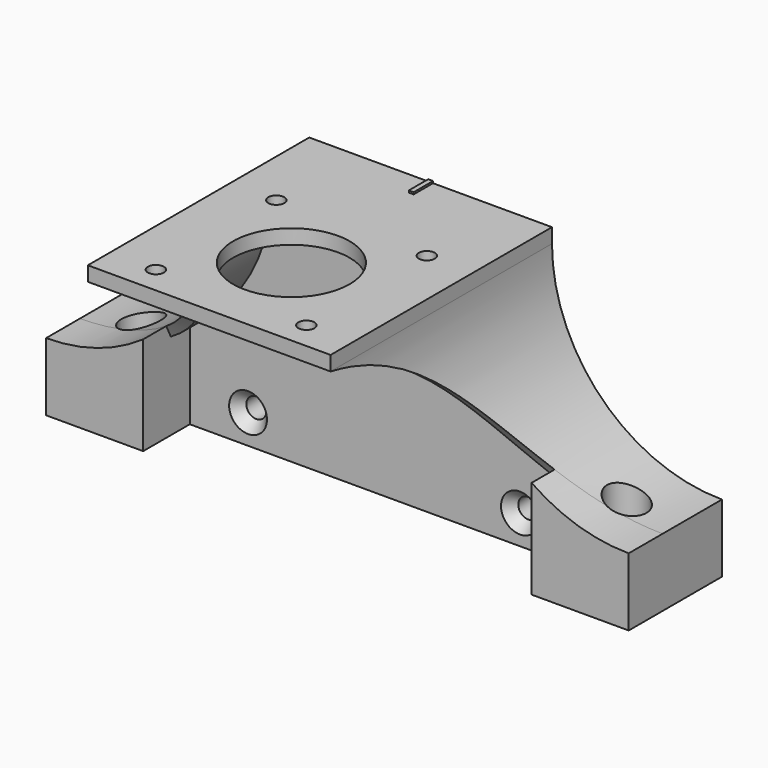
from build123d import *

# Parameters (mm, degrees)
F0_W           = 50
F0_H           = 3
F1_DEPTH       = 12
F3_DEPTH       = 45
F5_DEPTH       = 120.001
F6_R           = 12
F6_R_2         = 1.65
F7_DEPTH       = 25
F9_D           = 4.1000000042
F9_CSINK_D     = 7.7978
F9_CSINK_ANGLE = 82
F10_W          = 1
F10_H          = 5
F11_DEPTH      = 0.4
F13_END_RADIUS = 35
F13_REACH      = 75.7248075794
F14_END_RADIUS = 35
F14_REACH      = 75.7248075794
F15_DEPTH      = 25


with BuildPart() as f1:
    # F0 (on Front) → F1 (new body)
    with BuildSketch(Plane.XZ):
        with BuildLine():
            Line((22.8227958083, 19.723181963), (-27.1772041917, 19.723181963))
            ThreePointArc((-27.1772041917, 19.723181963), (-37.4284668502, -5.0255553786), (-62.1772041917, -15.276818037))
            Line((-62.1772041917, -15.276818037), (-62.1772041917, -29.276818037))
            Line((-62.1772041917, -29.276818037), (57.8227958083, -29.276818037))
            Line((57.8227958083, -29.276818037), (57.8227958083, -15.276818037))
            ThreePointArc((57.8227958083, -15.276818037), (33.0740584668, -5.0255553786), (22.8227958083, 19.723181963))
        make_face()
        with Locations((-2.1772041917, 21.223181963)):
            Rectangle(F0_W, F0_H)
    extrude(amount=F1_DEPTH)

    # F2 (on face) → F3 (join)
    with BuildSketch(Plane.XZ.offset(12)):
        with BuildLine():
            Line((-25.1772041917, 19.723181963), (-27.1772041917, 19.723181963))
            ThreePointArc((-27.1772041917, 19.723181963), (-37.4284668502, -5.0255553786), (-62.1772041917, -15.276818037))
            Line((-62.1772041917, -15.276818037), (-62.1772041917, -29.276818037))
            Line((-62.1772041917, -29.276818037), (-60.1772041917, -29.276818037))
            Line((-60.1772041917, -29.276818037), (-60.1772041917, -17.2227244409))
            ThreePointArc((-60.1772041917, -17.2227244409), (-35.3164521546, -5.722839337), (-25.1772041917, 19.723181963))
        make_face()
        Polygon((-27.1772041917, 22.723181963), (-27.1772041917, 19.723181963), (-25.1772041917, 19.723181963), (20.8227958083, 19.723181963), (22.8227958083, 19.723181963), (22.8227958083, 22.723181963), align=None)
        with BuildLine():
            Line((22.8227958083, 19.723181963), (20.8227958083, 19.723181963))
            ThreePointArc((20.8227958083, 19.723181963), (30.9620437712, -5.722839337), (55.8227958083, -17.2227244409))
            Line((55.8227958083, -17.2227244409), (55.8227958083, -29.276818037))
            Line((55.8227958083, -29.276818037), (57.8227958083, -29.276818037))
            Line((57.8227958083, -29.276818037), (57.8227958083, -15.276818037))
            ThreePointArc((57.8227958083, -15.276818037), (33.0740584668, -5.0255553786), (22.8227958083, 19.723181963))
        make_face()
    extrude(amount=F3_DEPTH)

    # F4 (on face) → F5 (cut, through all)
    with BuildSketch(Plane(origin=(-62.1772041917, 0, 0), x_dir=(0, -1, 0), z_dir=(-1, 0, 0))):
        with BuildLine():
            Line((57, -15.276818037), (57, 19.723181963))
            ThreePointArc((57, 19.723181963), (26.3280584166, 2.7280262742), (12, -29.276818037))
            Line((12, -29.276818037), (57, -29.276818037))
            Line((57, -29.276818037), (57, -15.276818037))
        make_face()
    extrude(amount=-F5_DEPTH, mode=Mode.SUBTRACT)

    # F6 (on face) → F7 (cut)
    with BuildSketch(Plane.XY.offset(22.723181963)):
        with Locations((-2.1772041917, -35.85)):
            Circle(F6_R)
        with Locations((-17.6772041917, -51.35)):
            Circle(F6_R_2)
        with Locations((-17.6772041917, -20.35)):
            Circle(F6_R_2)
        with Locations((13.3227958083, -51.35)):
            Circle(F6_R_2)
        with Locations((13.3227958083, -20.35)):
            Circle(F6_R_2)
    extrude(amount=-F7_DEPTH, mode=Mode.SUBTRACT)

    # F9 (through all)
    with Locations(Plane.XZ.offset(12)):
        with Locations((-30.1772041917, -23.2497712389), (25.8227958083, -23.2497712389)):
            CounterSinkHole(F9_D / 2, F9_CSINK_D / 2, counter_sink_angle=F9_CSINK_ANGLE)

    # F10 (on face) → F11 (join)
    with BuildSketch(Plane.XY.offset(22.723181963)):
        with Locations((-2.1772041917, -2.5)):
            Rectangle(F10_W, F10_H)
    extrude(amount=F11_DEPTH)

    f13_end = (Plane(origin=(-62.1772041917, -28.5, 19.723181963), x_dir=(0, 0, 1), z_dir=(0, 1, 0)) * Cylinder(F13_END_RADIUS, 437.0700631752, mode=Mode.PRIVATE)).faces().sort_by_distance((-37.4284668502, -0.7549172174, -5.0255553786))[0]
    # F12 (on face) → F13 (join, up to the whole of a round face its end follows)
    with BuildSketch(Plane(origin=(0, 0, -29.276818037), x_dir=(1, 0, 0), z_dir=(0, 0, -1))):
        with BuildLine():
            Line((-62.1772041917, 24), (-62.1772041917, 12))
            Line((-62.1772041917, 12), (-60.1772041917, 12))
            Line((-60.1772041917, 12), (-56.2272041917, 12))
            ThreePointArc((-56.2272041917, 12), (-52.1772041917, 16.05), (-48.1272041917, 12))
            Line((-48.1272041917, 12), (-42.1772041917, 12))
            Line((-42.1772041917, 12), (-42.1772041917, 24))
            Line((-42.1772041917, 24), (-62.1772041917, 24))
        make_face()
        with BuildLine():
            Line((-56.2272041917, 12), (-48.1272041917, 12))
            ThreePointArc((-48.1272041917, 12), (-52.1772041917, 16.05), (-56.2272041917, 12))
        make_face()
    f13_long = extrude(amount=-F13_REACH, mode=Mode.PRIVATE)
    add(split(f13_long, bisect_by=f13_end, keep=Keep.TOP, mode=Mode.PRIVATE))

    f14_end = (Plane(origin=(57.8227958083, -28.5, 19.723181963), x_dir=(0, 0, 1), z_dir=(0, 1, 0)) * Cylinder(F14_END_RADIUS, 437.0700631752, mode=Mode.PRIVATE)).faces().sort_by_distance((33.0740584668, -0.7549172174, -5.0255553786))[0]
    # F12 (on face) → F14 (join, up to the whole of a round face its end follows)
    with BuildSketch(Plane(origin=(0, 0, -29.276818037), x_dir=(1, 0, 0), z_dir=(0, 0, -1))):
        with BuildLine():
            Line((37.8227958083, 24), (37.8227958083, 12))
            Line((37.8227958083, 12), (43.7727958083, 12))
            ThreePointArc((43.7727958083, 12), (47.8227958083, 16.05), (51.8727958083, 12))
            Line((51.8727958083, 12), (55.8227958083, 12))
            Line((55.8227958083, 12), (57.8227958083, 12))
            Line((57.8227958083, 12), (57.8227958083, 24))
            Line((57.8227958083, 24), (37.8227958083, 24))
        make_face()
        with BuildLine():
            Line((51.8727958083, 12), (43.7727958083, 12))
            ThreePointArc((43.7727958083, 12), (47.8227958083, 7.95), (51.8727958083, 12))
        make_face()
    f14_long = extrude(amount=-F14_REACH, mode=Mode.PRIVATE)
    add(split(f14_long, bisect_by=f14_end, keep=Keep.TOP, mode=Mode.PRIVATE))

    # F12 (on face) → F15 (cut)
    with BuildSketch(Plane(origin=(0, 0, -29.276818037), x_dir=(1, 0, 0), z_dir=(0, 0, -1))):
        with BuildLine():
            Line((-56.2272041917, 12), (-48.1272041917, 12))
            ThreePointArc((-48.1272041917, 12), (-52.1772041917, 16.05), (-56.2272041917, 12))
        make_face()
        with BuildLine():
            ThreePointArc((-56.2272041917, 12), (-52.1772041917, 7.95), (-48.1272041917, 12))
            Line((-48.1272041917, 12), (-56.2272041917, 12))
        make_face()
        with BuildLine():
            Line((51.8727958083, 12), (43.7727958083, 12))
            ThreePointArc((43.7727958083, 12), (47.8227958083, 7.95), (51.8727958083, 12))
        make_face()
        with BuildLine():
            ThreePointArc((51.8727958083, 12), (47.8227958083, 16.05), (43.7727958083, 12))
            Line((43.7727958083, 12), (51.8727958083, 12))
        make_face()
    extrude(amount=-F15_DEPTH, mode=Mode.SUBTRACT)


solid = f1.part
